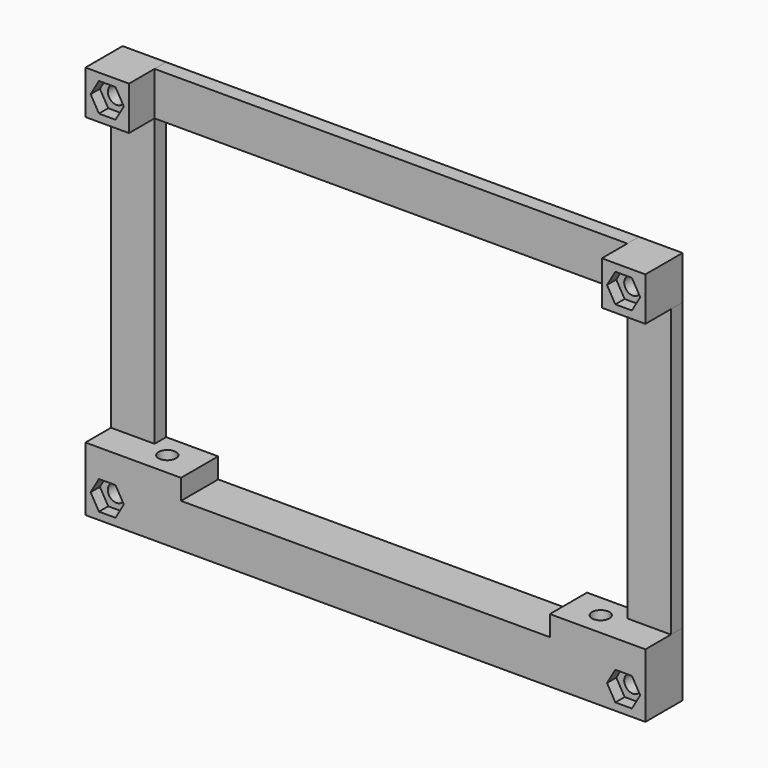
from build123d import *

# Parameters (mm, degrees)
F0_W     = 15
F0_H     = 15
F1_DEPTH = 16
F0_H_2   = 7
F0_W_2   = 17.9
F0_R     = 3
F2_DEPTH = 12
F0_H_3   = 98.65
F3_DEPTH = 5
F0_W_3   = 162.8
F6_D     = 6


with BuildPart() as f1:
    # F0 (on Front) → F1 (new body)
    with BuildSketch(Plane.XZ):
        with Locations((-88.9, 60.325)):
            Rectangle(F0_W, F0_H)
        Polygon((-83.184232335, 60.325), (-86.0421161675, 55.375), (-91.7578838325, 55.375), (-94.615767665, 60.325), (-91.7578838325, 65.275), (-86.0421161675, 65.275), align=None, mode=Mode.SUBTRACT)
    extrude(amount=F1_DEPTH)


with BuildPart() as f1b:
    # F0 (on Front) → F1, piece 2 (new body)
    with BuildSketch(Plane.XZ):
        with Locations((88.9, 60.325)):
            Rectangle(F0_W, F0_H)
        Polygon((94.615767665, 60.325), (91.7578838325, 55.375), (86.0421161675, 55.375), (83.184232335, 60.325), (86.0421161675, 65.275), (91.7578838325, 65.275), align=None, mode=Mode.SUBTRACT)
    extrude(amount=F1_DEPTH)


with BuildPart() as f1c:
    # F0 (on Front) → F1, piece 3 (new body)
    with BuildSketch(Plane.XZ):
        with Locations((-88.9, -49.325)):
            Rectangle(F0_W, F0_H_2)
        with Locations((-72.45, -49.325)):
            Rectangle(F0_W_2, F0_H_2)
        Polygon((-81.4, -52.825), (-96.4, -52.825), (-96.4, -67.825), (-85.725, -67.825), (-81.4, -67.825), align=None)
        Polygon((-94.615767665, -60.325), (-91.7578838325, -55.375), (-86.0421161675, -55.375), (-83.184232335, -60.325), (-86.0421161675, -65.275), (-91.7578838325, -65.275), align=None, mode=Mode.SUBTRACT)
        Polygon((-63.5, -52.825), (-81.4, -52.825), (-81.4, -67.825), (-63.5, -67.825), (63.5, -67.825), (70.725, -67.825), (81.4, -67.825), (81.4, -52.825), (63.5, -52.825), align=None)
        with Locations((88.9, -49.325)):
            Rectangle(F0_W, F0_H_2)
        with Locations((72.45, -49.325)):
            Rectangle(F0_W_2, F0_H_2)
        Polygon((96.4, -52.825), (81.4, -52.825), (81.4, -67.825), (85.725, -67.825), (96.4, -67.825), align=None)
        Polygon((83.184232335, -60.325), (86.0421161675, -55.375), (91.7578838325, -55.375), (94.615767665, -60.325), (91.7578838325, -65.275), (86.0421161675, -65.275), align=None, mode=Mode.SUBTRACT)
    extrude(amount=F1_DEPTH)

    # F0 (on Front) → F2 (join)
    with BuildSketch(Plane.XZ):
        Polygon((-86.0421161675, -55.375), (-91.7578838325, -55.375), (-94.615767665, -60.325), (-91.7578838325, -65.275), (-86.0421161675, -65.275), (-83.184232335, -60.325), align=None)
        with Locations((-88.9, -60.325)):
            Circle(F0_R, mode=Mode.SUBTRACT)
        Polygon((91.7578838325, -55.375), (86.0421161675, -55.375), (83.184232335, -60.325), (86.0421161675, -65.275), (91.7578838325, -65.275), (94.615767665, -60.325), align=None)
        with Locations((88.9, -60.325)):
            Circle(F0_R, mode=Mode.SUBTRACT)
    extrude(amount=F2_DEPTH)

    # F6 (through all)
    with Locations(Plane(origin=(0, 0, -67.825), x_dir=(1, 0, 0), z_dir=(0, 0, -1))):
        with Locations((74.6125, 8), (-74.6125, 8)):
            Hole(F6_D / 2)


with BuildPart() as f2:
    # F0 (on Front) → F2, piece 2 (new body)
    with BuildSketch(Plane.XZ):
        Polygon((-91.7578838325, 55.375), (-86.0421161675, 55.375), (-83.184232335, 60.325), (-86.0421161675, 65.275), (-91.7578838325, 65.275), (-94.615767665, 60.325), align=None)
        with Locations((-88.9, 60.325)):
            Circle(F0_R, mode=Mode.SUBTRACT)
    extrude(amount=F2_DEPTH)


with BuildPart() as f2b:
    # F0 (on Front) → F2, piece 3 (new body)
    with BuildSketch(Plane.XZ):
        Polygon((86.0421161675, 55.375), (91.7578838325, 55.375), (94.615767665, 60.325), (91.7578838325, 65.275), (86.0421161675, 65.275), (83.184232335, 60.325), align=None)
        with Locations((88.9, 60.325)):
            Circle(F0_R, mode=Mode.SUBTRACT)
    extrude(amount=F2_DEPTH)


with BuildPart() as f3:
    # F0 (on Front) → F3 (new body)
    with BuildSketch(Plane.XZ):
        with Locations((-88.9, 3.5)):
            Rectangle(F0_W, F0_H_3)
    extrude(amount=F3_DEPTH)


with BuildPart() as f3b:
    # F0 (on Front) → F3, piece 2 (new body)
    with BuildSketch(Plane.XZ):
        with Locations((0, 60.325)):
            Rectangle(F0_W_3, F0_H)
    extrude(amount=F3_DEPTH)


with BuildPart() as f3c:
    # F0 (on Front) → F3, piece 3 (new body)
    with BuildSketch(Plane.XZ):
        with Locations((88.9, 3.5)):
            Rectangle(F0_W, F0_H_3)
    extrude(amount=F3_DEPTH)


solid = Compound([f1.part, f1b.part, f1c.part, f2.part, f2b.part, f3.part, f3b.part, f3c.part])
